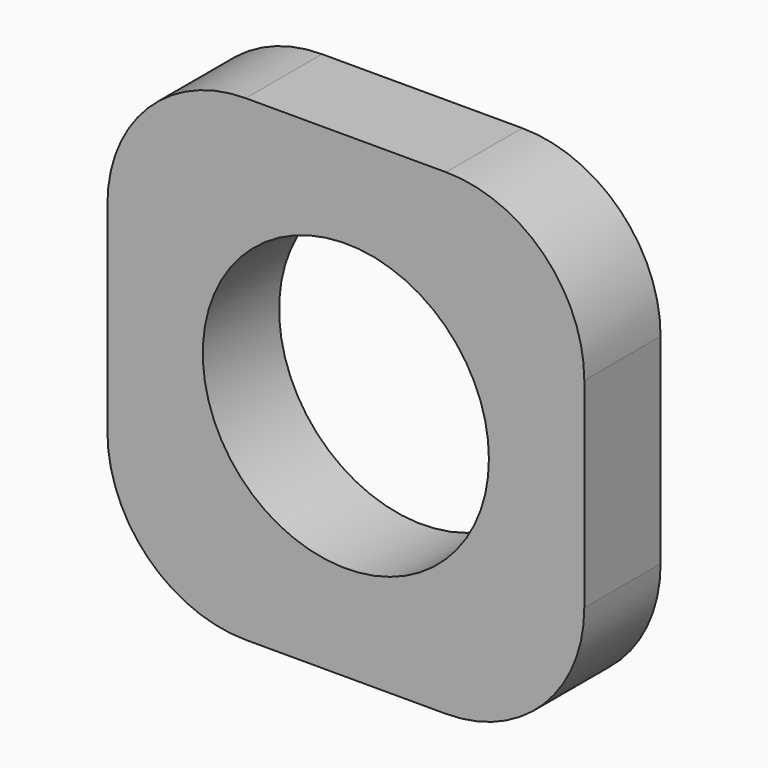
from build123d import *

# Parameters (mm, degrees)
F0_R     = 38.1
F2_DEPTH = 25.4
F3_DEPTH = 25.4
F4_DEPTH = 25.4


# Not quite as in the source:
# - the program builds the solid bodies; features that only make, move or delete a surface that nothing else refers to are left out


with BuildPart() as f2:
    # F0 (on Front) → F2 (new body)
    with BuildSketch(Plane.XZ):
        with BuildLine():
            Line((26.67, 63.5), (-26.6751700985, 63.5))
            ThreePointArc((-26.6751700985, 63.5), (-52.7142570379, 52.7142570379), (-63.5, 26.6751700985))
            Line((-63.5, 26.6751700985), (-63.5, -26.67))
            ThreePointArc((-63.5, -26.67), (-52.7127427511, -52.7127427511), (-26.67, -63.5))
            Line((-26.67, -63.5), (26.6751700985, -63.5))
            ThreePointArc((26.6751700985, -63.5), (52.7142570379, -52.7142570379), (63.5, -26.6751700985))
            Line((63.5, -26.6751700985), (63.5, 26.67))
            ThreePointArc((63.5, 26.67), (52.7127427511, 52.7127427511), (26.67, 63.5))
        make_face()
        Circle(F0_R, mode=Mode.SUBTRACT)
    extrude(amount=F2_DEPTH)


with BuildPart() as f3:
    # F0 (on Front) → F3 (new body)
    with BuildSketch(Plane.XZ):
        with BuildLine():
            Line((26.67, 63.5), (-26.6751700985, 63.5))
            ThreePointArc((-26.6751700985, 63.5), (-52.7142570379, 52.7142570379), (-63.5, 26.6751700985))
            Line((-63.5, 26.6751700985), (-63.5, -26.67))
            ThreePointArc((-63.5, -26.67), (-52.7127427511, -52.7127427511), (-26.67, -63.5))
            Line((-26.67, -63.5), (26.6751700985, -63.5))
            ThreePointArc((26.6751700985, -63.5), (52.7142570379, -52.7142570379), (63.5, -26.6751700985))
            Line((63.5, -26.6751700985), (63.5, 26.67))
            ThreePointArc((63.5, 26.67), (52.7127427511, 52.7127427511), (26.67, 63.5))
        make_face()
        Circle(F0_R, mode=Mode.SUBTRACT)
    extrude(amount=F3_DEPTH)


with BuildPart() as f4:
    # F0 (on Front) → F4 (new body)
    with BuildSketch(Plane.XZ):
        with BuildLine():
            Line((26.67, 63.5), (-26.6751700985, 63.5))
            ThreePointArc((-26.6751700985, 63.5), (-52.7142570379, 52.7142570379), (-63.5, 26.6751700985))
            Line((-63.5, 26.6751700985), (-63.5, -26.67))
            ThreePointArc((-63.5, -26.67), (-52.7127427511, -52.7127427511), (-26.67, -63.5))
            Line((-26.67, -63.5), (26.6751700985, -63.5))
            ThreePointArc((26.6751700985, -63.5), (52.7142570379, -52.7142570379), (63.5, -26.6751700985))
            Line((63.5, -26.6751700985), (63.5, 26.67))
            ThreePointArc((63.5, 26.67), (52.7127427511, 52.7127427511), (26.67, 63.5))
        make_face()
        Circle(F0_R, mode=Mode.SUBTRACT)
    extrude(amount=F4_DEPTH)


solid = Compound([f2.part, f3.part, f4.part])
